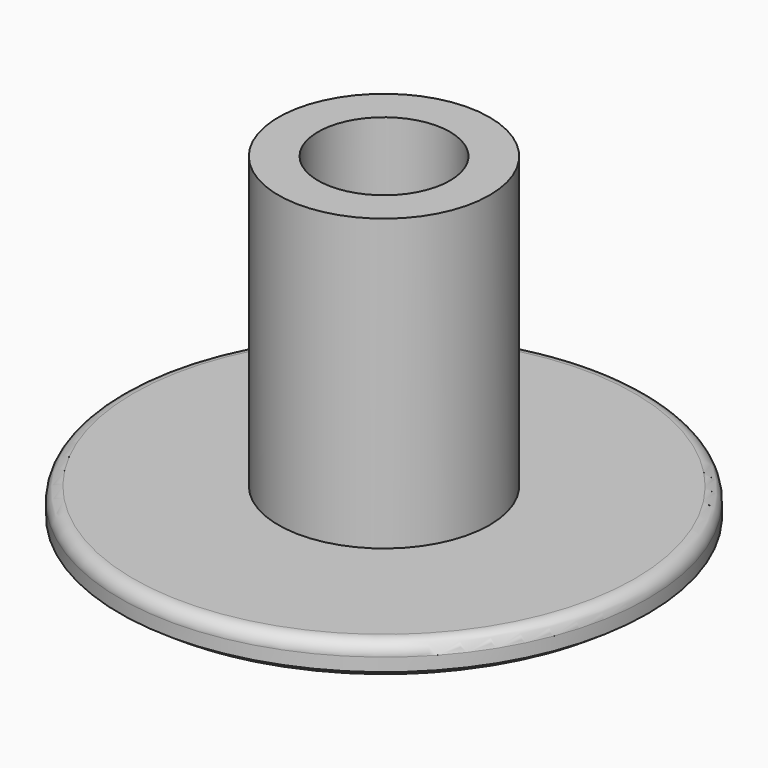
from build123d import *

# Parameters (mm, degrees)
F0_R     = 10
F0_R_2   = 4
F1_DEPTH = 2
F0_R_3   = 2.5
F2_DEPTH = 11
F3_R     = 0.5
F4_DEPTH = 2
F5_SIZE  = 1


# Not quite as in the source:
# - a fillet or chamfer that OpenCascade refuses, or shapes differently, is made with other operations: its cross-section is extruded or revolved along the edge and cut away or added


with BuildPart() as f1:
    # F0 (on Top) → F1 (new body)
    with BuildSketch(Plane.XY):
        Circle(F0_R)
        Circle(F0_R_2, mode=Mode.SUBTRACT)
    extrude(amount=-F1_DEPTH)

    # F3
    f3_edges = [f1.edges().sort_by_distance(p)[0] for p in [
        (-10, 0, 0),
    ]]
    fillet(f3_edges, radius=F3_R)

    # F5
    f5_edges = [f1.edges().sort_by_distance(p)[0] for p in [
        (-10, 0, -2),
    ]]
    chamfer(f5_edges, length=F5_SIZE)

    # F6: fillet of radius 5 on 1 edges, made by hand

    # F6_s1 → F6_t2 (revolve, cut)
    with BuildSketch(Plane.XZ):
        with BuildLine():
            ThreePointArc((10, -1), (8.5811388301, -1.7434164903), (7, -2))
            Line((7, -2), (9, -2))
            Line((9, -2), (10, -1))
        make_face()
    revolve(axis=Axis((0, 0, -2), (0, 0, 1)), mode=Mode.SUBTRACT)


with BuildPart() as f2:
    # F0 (on Top) → F2 (new body)
    with BuildSketch(Plane.XY):
        Circle(F0_R_2)
        Circle(F0_R_3, mode=Mode.SUBTRACT)
    extrude(amount=F2_DEPTH)


with BuildPart() as f4:
    # F0 (on Top) → F4 (new body)
    with BuildSketch(Plane.XY):
        Circle(F0_R_2)
        Circle(F0_R_3, mode=Mode.SUBTRACT)
    extrude(amount=-F4_DEPTH)


solid = Compound([f1.part, f2.part, f4.part])
